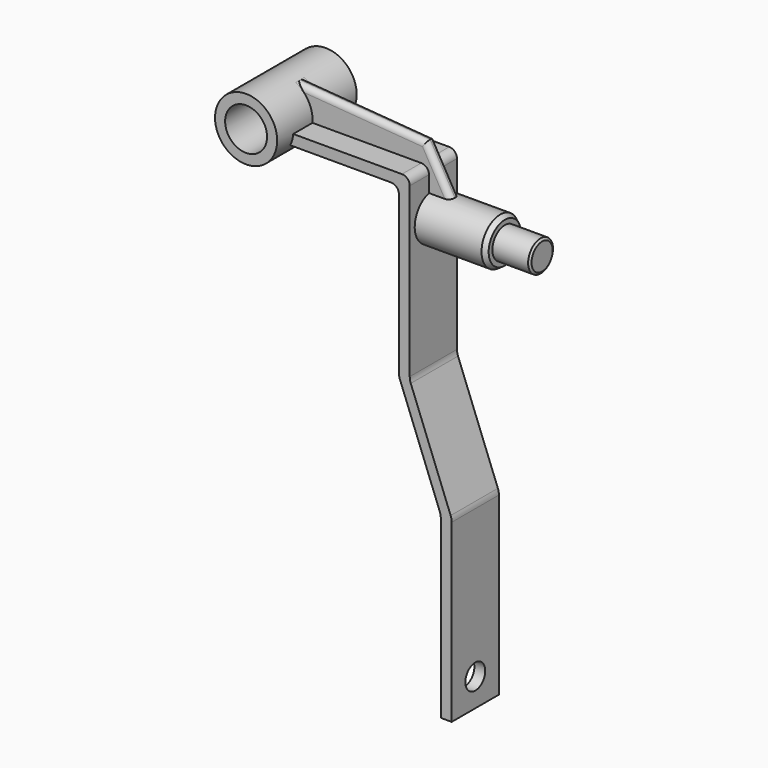
from build123d import *

# Parameters (mm, degrees)
F0_R           = 13.5
F1_DEPTH       = 64
F2_W           = 102
F2_H           = 13
F3_DEPTH       = 400
F5_DEPTH       = 13
F7_DEPTH       = 13
F8_R           = 15
F9_DEPTH       = 43
F14_DEPTH      = 3.5
F14_DEPTH_BACK = 3.5
F15_R          = 8
F16_DEPTH      = 25
F17_T4_DEPTH   = 101.551131953
F17_S5_R       = 20
F17_T6_DEPTH   = 53
F17_T10_DEPTH  = 101.551131953
F17_S11_R      = 20
F17_T12_DEPTH  = 53
F17_T16_DEPTH  = 50.1219672703
F17_S17_R      = 15
F17_T18_DEPTH  = 28
F17_T22_DEPTH  = 50.1219672703
F17_S23_R      = 15
F17_T24_DEPTH  = 28


# Not quite as in the source:
# - a fillet or chamfer that OpenCascade refuses, or shapes differently, is made with other operations: its cross-section is extruded or revolved along the edge and cut away or added


with BuildPart() as f1:
    # F0 (on Front) → F1 (new body)
    with BuildSketch(Plane.XZ):
        with BuildLine():
            Line((-7, -214.9833835959), (0, -214.9833835959))
            Line((0, -214.9833835959), (0, -101.8451102358))
            ThreePointArc((0, -101.8451102358), (-0.1689225963, -100.0148323657), (-0.6699834164, -98.2463895535))
            Line((-0.6699834164, -98.2463895535), (-26.3300165836, -31.7203776383))
            ThreePointArc((-26.3300165836, -31.7203776383), (-26.8310774037, -29.9519348262), (-27, -28.1216569561))
            Line((-27, -28.1216569561), (-27, 80.0166164041))
            ThreePointArc((-27, 80.0166164041), (-28.4644660941, 83.55215031), (-32, 85.0166164041))
            Line((-32, 85.0166164041), (-102, 85.0166164041))
            ThreePointArc((-102, 85.0166164041), (-141.2677104995, 91.7114873793), (-103.8614958525, 78.0166164041))
            Line((-103.8614958525, 78.0166164041), (-39, 78.0166164041))
            ThreePointArc((-39, 78.0166164041), (-35.4644660941, 76.55215031), (-34, 73.0166164041))
            Line((-34, 73.0166164041), (-34, -28.1216569561))
            ThreePointArc((-34, -28.1216569561), (-33.8310774037, -29.9519348262), (-33.3300165836, -31.7203776383))
            Line((-33.3300165836, -31.7203776383), (-7.6699834164, -98.2463895535))
            ThreePointArc((-7.6699834164, -98.2463895535), (-7.1689225963, -100.0148323657), (-7, -101.8451102358))
            Line((-7, -101.8451102358), (-7, -214.9833835959))
        make_face()
        with Locations((-121.9394617303, 86.5715652479)):
            Circle(F0_R, mode=Mode.SUBTRACT)
    extrude(amount=F1_DEPTH)

    # F2 (on face) → F3 (cut)
    with BuildSketch(Plane.XY.offset(85.0166164041)):
        with Locations((-51, -6.5)):
            Rectangle(F2_W, F2_H)
        with Locations((-51, -57.5)):
            Rectangle(F2_W, F2_H)
    extrude(amount=-F3_DEPTH, mode=Mode.SUBTRACT)

    # F4 (on face) → F5 (cut)
    with BuildSketch(Plane(origin=(0, 0, 0), x_dir=(-1, 0, 0), z_dir=(0, 1, 0))):
        with BuildLine():
            ThreePointArc((103.8614958525, 78.0166164041), (102.6112129611, 81.4316431166), (102, 85.0166164041))
            Line((102, 85.0166164041), (102, 78.0166164041))
            Line((102, 78.0166164041), (103.8614958525, 78.0166164041))
        make_face()
    extrude(amount=-F5_DEPTH, mode=Mode.SUBTRACT)

    # F6 (on face) → F7 (cut)
    with BuildSketch(Plane.XZ.offset(64)):
        with BuildLine():
            Line((-102, 78.0166164041), (-102, 85.0166164041))
            ThreePointArc((-102, 85.0166164041), (-102.6112129611, 81.4316431166), (-103.8614958525, 78.0166164041))
            Line((-103.8614958525, 78.0166164041), (-102, 78.0166164041))
        make_face()
    extrude(amount=-F7_DEPTH, mode=Mode.SUBTRACT)

    # F8 (on face) → F9 (join)
    with BuildSketch(Plane.YZ.offset(-27)):
        with Locations((-32, 55.0166164041)):
            Circle(F8_R)
    extrude(amount=F9_DEPTH)

    # F11 (on face) → F12 (revolve)
    with BuildSketch(Plane(origin=(0, -32, 0), x_dir=(-1, 0, 0), z_dir=(0, 1, 0))):
        Polygon((-16, 55.0166164041), (-16, 70.0166164041), (-19, 68.0166164041), (-19, 65.0166164041), (-42, 65.0166164041), (-43, 63.5166164041), (-43, 55.0166164041), align=None)
    revolve(axis=Axis((29.5, -32, 55.0166164041), (1, 0, 0)))

    # F13 (on face) → F14 (join, two sides)
    with BuildSketch(Plane(origin=(0, -32, 0), x_dir=(-1, 0, 0), z_dir=(0, 1, 0))) as f14_sk:
        with BuildLine():
            ThreePointArc((102.0563293248, 85.0166164041), (104.6045567862, 96.385687049), (113.0563293248, 104.4054608288))
            Line((113.0563293248, 104.4054608288), (29.0563293248, 97.8962504797))
            Line((29.0563293248, 97.8962504797), (13.0563293248, 70.0166164041))
            Line((13.0563293248, 70.0166164041), (10.7852649025, 66.0593385881))
            Line((10.7852649025, 66.0593385881), (27, 66.0593385881))
            Line((27, 66.0593385881), (27, 70.0166164041))
            Line((27, 70.0166164041), (27, 80.0166164041))
            ThreePointArc((27, 80.0166164041), (28.4644660941, 83.55215031), (32, 85.0166164041))
            Line((32, 85.0166164041), (102.0563293248, 85.0166164041))
        make_face()
    extrude(amount=F14_DEPTH)
    extrude(f14_sk.sketch, amount=-F14_DEPTH_BACK)

    # F15 (on face) → F16 (cut)
    with BuildSketch(Plane.YZ):
        with Locations((-32, -196.9833835959)):
            Circle(F15_R)
    extrude(amount=-F16_DEPTH, mode=Mode.SUBTRACT)

    # F17: fillet of radius 3.5 on 4 edges, made by hand


with BuildPart() as f17_tool2:
    # F17_s3 → F17_t4 (new body)
    with BuildSketch(Plane(origin=(-128.9474066936, 0, 9.992211835), x_dir=(0, 1, 0), z_dir=(0.9970110578, 0, -0.0772589845))):
        with BuildLine():
            ThreePointArc((-35.5, 91.8587817466), (-34.4748737342, 94.3336554808), (-32, 95.3587817466))
            Line((-32, 95.3587817466), (-35.5, 95.3587817466))
            Line((-35.5, 95.3587817466), (-35.5, 91.8587817466))
        make_face()
    extrude(amount=F17_T4_DEPTH)

    # F17_s5 → F17_t6 (cut, symmetric)
    with BuildSketch(Plane.XZ.offset(33.8)):
        with Locations((-121.9394617303, 86.5715652479)):
            Circle(F17_S5_R)
    extrude(amount=F17_T6_DEPTH, both=True, mode=Mode.SUBTRACT)


with BuildPart() as f1_1:
    add(f1.part)

    # F17_t1: cut F17_tool2
    add(f17_tool2.part, mode=Mode.SUBTRACT)


with BuildPart() as f17_tool8:
    # F17_s9 → F17_t10 (new body)
    with BuildSketch(Plane(origin=(-128.9474066936, 0, 9.992211835), x_dir=(0, 1, 0), z_dir=(0.9970110578, 0, -0.0772589845))):
        with BuildLine():
            ThreePointArc((-28.5, 91.8587817466), (-29.5251262658, 94.3336554808), (-32, 95.3587817466))
            Line((-32, 95.3587817466), (-28.5, 95.3587817466))
            Line((-28.5, 95.3587817466), (-28.5, 91.8587817466))
        make_face()
    extrude(amount=F17_T10_DEPTH)

    # F17_s11 → F17_t12 (cut, symmetric)
    with BuildSketch(Plane.XZ.offset(30.2)):
        with Locations((-121.9394617303, 86.5715652479)):
            Circle(F17_S11_R)
    extrude(amount=F17_T12_DEPTH, both=True, mode=Mode.SUBTRACT)


with BuildPart() as f1_2:
    add(f1_1.part)

    # F17_t7: cut F17_tool8
    add(f17_tool8.part, mode=Mode.SUBTRACT)


with BuildPart() as f17_tool14:
    # F17_s15 → F17_t16 (new body)
    with BuildSketch(Plane(origin=(-53.8169429454, 0, 93.7747922742), x_dir=(0, 1, 0), z_dir=(0.4977511049, 0, -0.8673199165))):
        with BuildLine():
            ThreePointArc((-35.5, 20.026833714), (-34.4748737342, 22.5017074481), (-32, 23.526833714))
            Line((-32, 23.526833714), (-35.5, 23.526833714))
            Line((-35.5, 23.526833714), (-35.5, 20.026833714))
        make_face()
    extrude(amount=F17_T16_DEPTH)

    # F17_s17 → F17_t18 (cut, symmetric)
    with BuildSketch(Plane.YZ.offset(-22.5)):
        with Locations((-32, 55.0166164041)):
            Circle(F17_S17_R)
    extrude(amount=F17_T18_DEPTH, both=True, mode=Mode.SUBTRACT)


with BuildPart() as f1_3:
    add(f1_2.part)

    # F17_t13: cut F17_tool14
    add(f17_tool14.part, mode=Mode.SUBTRACT)


with BuildPart() as f17_tool20:
    # F17_s21 → F17_t22 (new body)
    with BuildSketch(Plane(origin=(-28.8686783585, 0, 50.3030118051), x_dir=(0, 1, 0), z_dir=(-0.4977511049, 0, 0.8673199165))):
        with BuildLine():
            ThreePointArc((-28.5, -20.026833714), (-29.5251262658, -22.5017074481), (-32, -23.526833714))
            Line((-32, -23.526833714), (-28.5, -23.526833714))
            Line((-28.5, -23.526833714), (-28.5, -20.026833714))
        make_face()
    extrude(amount=F17_T22_DEPTH)

    # F17_s23 → F17_t24 (cut, symmetric)
    with BuildSketch(Plane.YZ.offset(-22.5)):
        with Locations((-32, 55.0166164041)):
            Circle(F17_S23_R)
    extrude(amount=F17_T24_DEPTH, both=True, mode=Mode.SUBTRACT)


with BuildPart() as f1_4:
    add(f1_3.part)

    # F17_t19: cut F17_tool20
    add(f17_tool20.part, mode=Mode.SUBTRACT)


solid = f1_4.part
